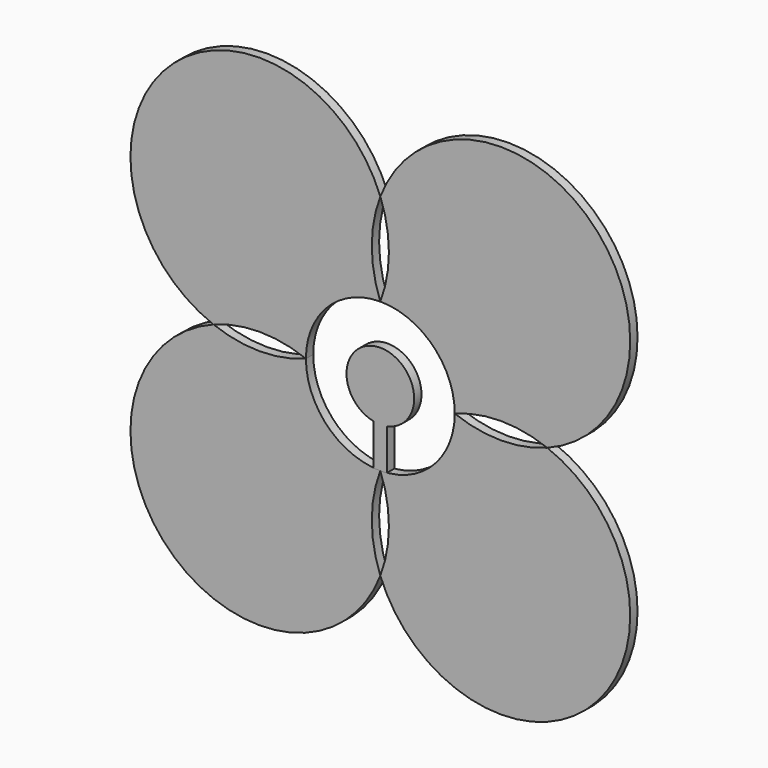
from build123d import *

# Parameters (mm, degrees)
F1_DEPTH = 0.254
F3_DEPTH = 0.254


with BuildPart() as f1:
    # F0 (on Front) → F1 (new body)
    with BuildSketch(Plane.XZ):
        with BuildLine():
            ThreePointArc((4.6260023192, 0), (3.3442261435, -0.2372258893), (2.0624499678, 0))
            ThreePointArc((2.0624499678, 0), (1.4583723581, -1.4583723581), (0, -2.0624499678))
            ThreePointArc((0, -2.0624499678), (0.2372258893, -3.3442261435), (0, -4.6260023192))
            ThreePointArc((0, -4.6260023192), (5.8766951624, -5.8766951624), (4.6260023192, 0))
        make_face()
    extrude(amount=F1_DEPTH)


with BuildPart() as f1b:
    # F0 (on Front) → F1, piece 2 (new body)
    with BuildSketch(Plane.XZ):
        with BuildLine():
            ThreePointArc((0, 2.0624499678), (1.4583723581, 1.4583723581), (2.0624499678, 0))
            ThreePointArc((2.0624499678, 0), (3.3442261435, 0.2372258893), (4.6260023192, 0))
            ThreePointArc((4.6260023192, 0), (5.8766951624, 5.8766951624), (0, 4.6260023192))
            ThreePointArc((0, 4.6260023192), (0.2372258893, 3.3442261435), (0, 2.0624499678))
        make_face()
    extrude(amount=F1_DEPTH)


with BuildPart() as f1c:
    # F0 (on Front) → F1, piece 3 (new body)
    with BuildSketch(Plane.XZ):
        with BuildLine():
            ThreePointArc((-2.0624499678, 0), (-1.4583723581, 1.4583723581), (0, 2.0624499678))
            ThreePointArc((0, 2.0624499678), (-0.2372258893, 3.3442261435), (0, 4.6260023192))
            ThreePointArc((0, 4.6260023192), (-5.8766951624, 5.8766951624), (-4.6260023192, 0))
            ThreePointArc((-4.6260023192, 0), (-3.3442261435, 0.2372258893), (-2.0624499678, 0))
        make_face()
    extrude(amount=F1_DEPTH)


with BuildPart() as f1d:
    # F0 (on Front) → F1, piece 4 (new body)
    with BuildSketch(Plane.XZ):
        with BuildLine():
            ThreePointArc((0, -4.6260023192), (-0.2372258893, -3.3442261435), (0, -2.0624499678))
            ThreePointArc((0, -2.0624499678), (-1.4583723581, -1.4583723581), (-2.0624499678, 0))
            ThreePointArc((-2.0624499678, 0), (-3.3442261435, -0.2372258893), (-4.6260023192, 0))
            ThreePointArc((-4.6260023192, 0), (-5.8766951624, -5.8766951624), (0, -4.6260023192))
        make_face()
    extrude(amount=F1_DEPTH)


with BuildPart() as f3:
    # F2 (on Front) → F3 (new body)
    with BuildSketch(Plane.XZ):
        with BuildLine():
            Line((0.1891683727, -2.0637542475), (0.1891683727, -0.918299452))
            ThreePointArc((0.1891683727, -0.918299452), (0, 0.9375812268), (-0.1891683727, -0.918299452))
            Line((-0.1891683727, -0.918299452), (-0.1891683727, -2.0637542475))
            Line((-0.1891683727, -2.0637542475), (0.1891683727, -2.0637542475))
        make_face()
    extrude(amount=F3_DEPTH)


solid = Compound([f1.part, f1b.part, f1c.part, f1d.part, f3.part])
